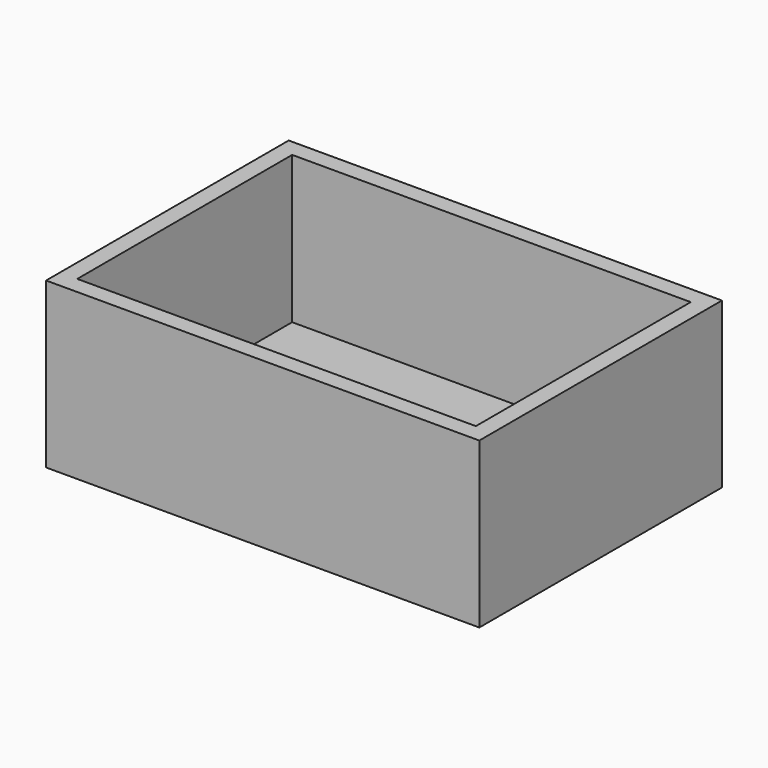
from build123d import *

# Parameters (mm, degrees)
F2_W     = 158.75
F2_H     = 111.125
F3_DEPTH = 6.35
F4_W     = 158.75
F4_H     = 111.125
F4_W_2   = 146.05
F4_H_2   = 98.425
F5_DEPTH = 53.975


# Not quite as in the source:
# - a length typed as a fraction of an inch, garbled in the dataset ("3 / 203.2 mm" for 3/8 in), is restored


with BuildPart() as f3:
    # F2 (on Top) → F3 (new body)
    with BuildSketch(Plane.XY):
        Rectangle(F2_W, F2_H)
    extrude(amount=F3_DEPTH)

    # F4 (on face) → F5 (join)
    with BuildSketch(Plane.XY.offset(6.35)):
        Rectangle(F4_W, F4_H)
        Rectangle(F4_W_2, F4_H_2, mode=Mode.SUBTRACT)
    extrude(amount=F5_DEPTH)


solid = f3.part
